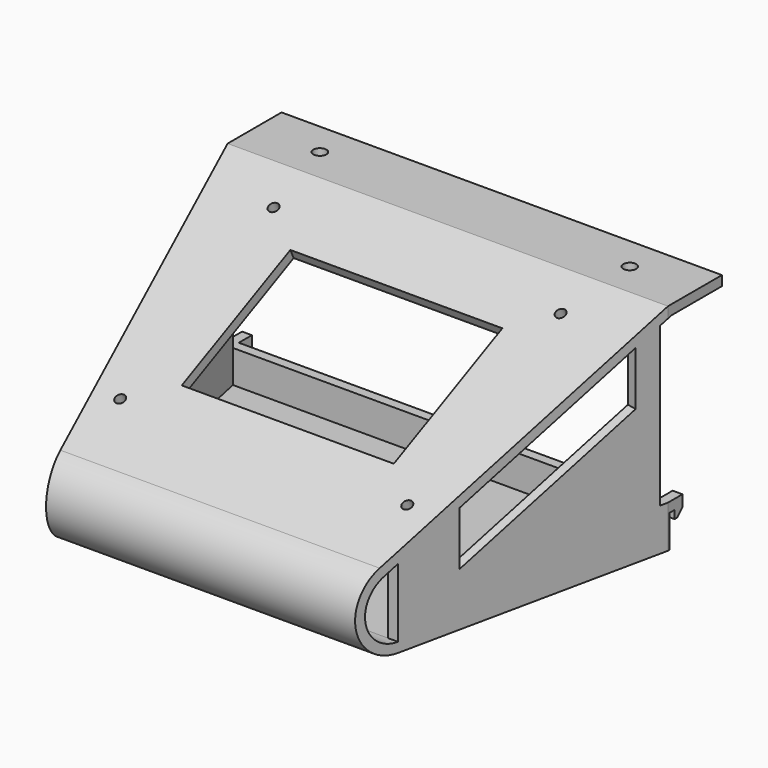
from build123d import *

# Parameters (mm, degrees)
F1_DEPTH       = 135
F2_R           = 1.5
F2_W           = 65
F2_H           = 46
F3_DEPTH       = 3
F4_R           = 2
F5_DEPTH       = 3
F6_SIZE        = 2
F7_R           = 5
F10_DEPTH      = 116
F15_DEPTH      = 64.5
F15_DEPTH_BACK = 64.5
F17_REACH      = 144.7359325659
F19_DEPTH      = 2.9344428022


# Not quite as in the source:
# - a feature names something its author has since deleted; it is built from what else it names


with BuildPart() as f1:
    # F0 (on Right) → F1 (new body)
    with BuildSketch(Plane.YZ):
        with BuildLine():
            Line((-106.670074853, -43.9587721159), (-20, -3))
            Line((-20, -3), (0, -3))
            Line((0, -3), (0, 0))
            Line((0, 0), (-20.6731804218, 0))
            Line((-20.6731804218, 0), (-107.9518930349, -41.2464037506))
            ThreePointArc((-107.9518930349, -41.2464037506), (-115.0819199271, -55.8463352542), (-102.3973475803, -66))
            Line((-102.3973475803, -66), (-20.1261255298, -66))
            Line((-20.1261255298, -66), (-20.1261255298, -56))
            Line((-20.1261255298, -56), (-18.1261255298, -56))
            Line((-18.1261255298, -56), (-18.1261255298, -58.5))
            Line((-18.1261255298, -58.5), (-15.1261255298, -58.5))
            Line((-15.1261255298, -58.5), (-15.1261255298, -53))
            Line((-15.1261255298, -53), (-23.1261255298, -53))
            Line((-23.1261255298, -53), (-23.1261255298, -63))
            Line((-23.1261255298, -63), (-102.3973475803, -63))
            ThreePointArc((-102.3973475803, -63), (-112.154710924, -55.189488657), (-106.670074853, -43.9587721159))
        make_face()
    extrude(amount=F1_DEPTH)

    # F2 (on face) → F3 (cut, through all)
    with BuildSketch(Plane(origin=(0, -3.7741368225, 7.9861945076), x_dir=(1, 0, 0), z_dir=(0, -0.4272727273, 0.9041227884))):
        with Locations((23, -31.0000917132)):
            Circle(F2_R)
        with Locations((111, -31.0000917132)):
            Circle(F2_R)
        with Locations((111, -96.0000917132)):
            Circle(F2_R)
        with Locations((23, -96.0000917132)):
            Circle(F2_R)
        with Locations((67.5, -63.5000917132)):
            Rectangle(F2_W, F2_H)
    extrude(amount=-F3_DEPTH, mode=Mode.SUBTRACT)

    # F4 (on face) → F5 (cut, through all)
    with BuildSketch(Plane.XY):
        with Locations((20, -10.3)):
            Circle(F4_R)
        with Locations((115, -10.3)):
            Circle(F4_R)
    extrude(amount=-F5_DEPTH, mode=Mode.SUBTRACT)

    # F6
    f6_edges = [f1.edges().sort_by_distance(p)[0] for p in [
        (67.5, -15.126126, -58.5),
    ]]
    chamfer(f6_edges, length=F6_SIZE)

    # F7
    f7_edges = [f1.edges().sort_by_distance(p)[0] for p in [
        (67.5, -20, -3),
    ]]
    fillet(f7_edges, radius=F7_R)

    # F9 (on offset) → F10 (cut, through all)
    with BuildSketch(Plane.XY.offset(50)):
        Polygon((26.5695702088, -145.6731804218), (0, -20.6731804218), (0, -145.6731804218), align=None)
        Polygon((135, -145.6731804218), (135, -20.6731804218), (108.4304297912, -145.6731804218), align=None)
    extrude(amount=-F10_DEPTH, mode=Mode.SUBTRACT)

    # F11 (on face) → F12 (join, up to the next surface of F1)
    with BuildSketch(Plane.XY.offset(-63)):
        Polygon((114.6289920234, -102.3973475803), (117.6289920234, -102.3973475803), (134.4786104219, -23.1261255298), (131.4786104219, -23.1261255298), align=None)
    extrude(until=Until.NEXT)

    # F14 (on offset) → F15 (cut, two sides)
    with BuildSketch(Plane.YZ.offset(67.5)) as f15_sk:
        Polygon((-15.1261255298, -53), (-20.1261255298, -53), (-20.1261255298, -56), (-18.1261255298, -56), (-18.1261255298, -58.5), (-17.1261255298, -58.5), (-15.1261255298, -56.5), align=None)
    extrude(amount=-F15_DEPTH, mode=Mode.SUBTRACT)
    extrude(f15_sk.sketch, amount=F15_DEPTH_BACK, mode=Mode.SUBTRACT)

    f17_end = f1.faces().sort_by_distance((10.9056419214, -64.0293542161, -20.4893747382))[0]
    # F16 (on face) → F17 (join, up to a face of the model that its end follows)
    with BuildSketch(Plane.XY.offset(-63)):
        Polygon((0.5213895781, -23.1261255298), (17.3710079766, -102.3973475803), (20.4380297612, -102.3973475803), (3.5884113627, -23.1261255298), align=None)
    f17_long = extrude(amount=F17_REACH, mode=Mode.PRIVATE)
    add(split(f17_long, bisect_by=f17_end, keep=Keep.BOTTOM, mode=Mode.PRIVATE))

    # F18 (on face) → F19 (cut, through all)
    with BuildSketch(Plane(origin=(133.3685883941, -28.3483685838, 0), x_dir=(0.2079116908, 0.9781476007, 0), z_dir=(0.9781476007, -0.2079116908, 0))):
        Polygon((-2.1533435687, -7.9275703375), (-56.6160369654, -33.1032536049), (-56.6160369654, -49.6283268957), (-2.1533435687, -24.4526436284), align=None)
    extrude(amount=-F19_DEPTH, mode=Mode.SUBTRACT)


solid = f1.part
